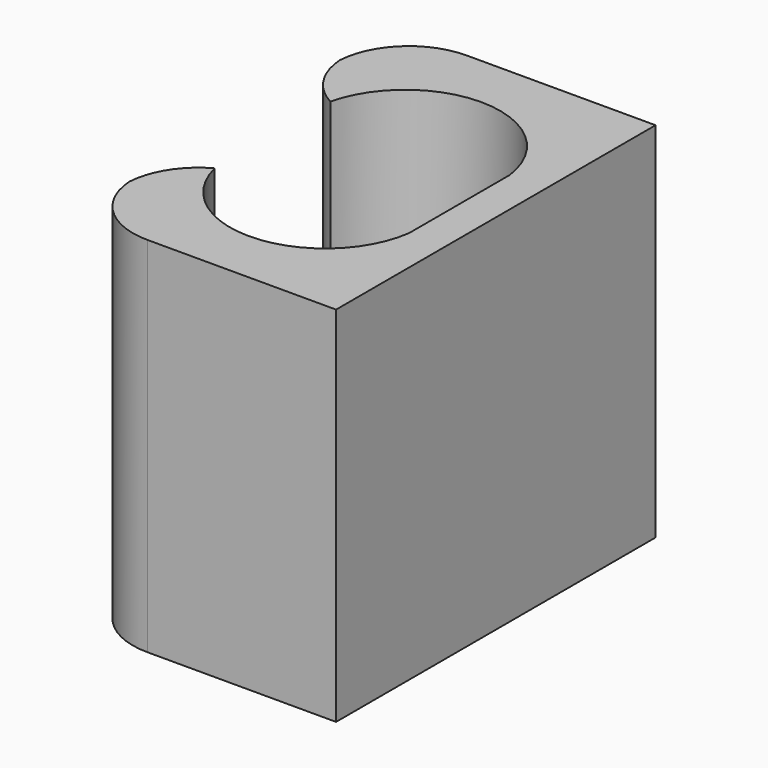
from build123d import *

# Parameters (mm, degrees)
F1_DEPTH    = 10
F2_DEPTH    = 5
F3_T1_DEPTH = 20


# Not quite as in the source:
# - a fillet or chamfer that OpenCascade refuses, or shapes differently, is made with other operations: its cross-section is extruded or revolved along the edge and cut away or added


with BuildPart() as f1:
    # F0 (on Top) → F1 (new body)
    with BuildSketch(Plane.XY):
        with BuildLine():
            ThreePointArc((-2.8424912948, 2.0151155274), (-0.2360435678, 4.2655420814), (2.3550239983, 1.9974242942))
            Line((2.3550239983, 1.9974242942), (2.3550239983, -1.4671932394))
            ThreePointArc((2.3550239983, -1.4671932394), (-0.2360435678, -3.7353110266), (-2.8424912948, -1.4848844726))
            Line((-2.8424912948, -1.4848844726), (-3.8449760017, -1.4848844726))
            Line((-3.8449760017, -1.4848844726), (-3.8449760017, -5.2353262286))
            Line((-3.8449760017, -5.2353262286), (3.3550239983, -5.2353262286))
            Line((3.3550239983, -5.2353262286), (3.3550239983, 5.7655572834))
            Line((3.3550239983, 5.7655572834), (-3.8449760017, 5.7655572834))
            Line((-3.8449760017, 5.7655572834), (-3.8449760017, 2.0151155274))
            Line((-3.8449760017, 2.0151155274), (-2.8424912948, 2.0151155274))
        make_face()
    extrude(amount=F1_DEPTH)

    # F0 (on Top) → F2 (join)
    with BuildSketch(Plane.XY):
        with BuildLine():
            Line((2.3550239983, -1.4671932394), (2.3550239983, 1.9974242942))
            ThreePointArc((2.3550239983, 1.9974242942), (-0.2360435678, 4.2655420814), (-2.8424912948, 2.0151155274))
            Line((-2.8424912948, 2.0151155274), (-1.4057946783, 2.0151155274))
            ThreePointArc((-1.4057946783, 2.0151155274), (0.7480700142, 2.1154829532), (1.8550239983, 0.2651155274))
            ThreePointArc((1.8550239983, 0.2651155274), (0.7480700142, -1.5852518984), (-1.4057946783, -1.4848844726))
            Line((-1.4057946783, -1.4848844726), (-2.8424912948, -1.4848844726))
            ThreePointArc((-2.8424912948, -1.4848844726), (-0.2360435678, -3.7353110266), (2.3550239983, -1.4671932394))
        make_face()
    extrude(amount=F2_DEPTH)

    # F3: fillet of radius 2 on 4 edges, made by hand

    # F3_s2 → F3_t1 (cut)
    with BuildSketch(Plane.XY.offset(-5)):
        with BuildLine():
            ThreePointArc((-1.8449760017, 2.0151155274), (-3.259189564, 2.600901965), (-3.8449760017, 4.0151155274))
            Line((-3.8449760017, 4.0151155274), (-3.8449760017, 2.0151155274))
            Line((-3.8449760017, 2.0151155274), (-1.8449760017, 2.0151155274))
        make_face()
        with BuildLine():
            ThreePointArc((-1.8449760017, -1.4848844726), (-3.259189564, -2.0706709102), (-3.8449760017, -3.4848844726))
            Line((-3.8449760017, -3.4848844726), (-3.8449760017, -1.4848844726))
            Line((-3.8449760017, -1.4848844726), (-1.8449760017, -1.4848844726))
        make_face()
        with BuildLine():
            ThreePointArc((-1.8449760017, -5.2353262286), (-3.259189564, -4.6495397909), (-3.8449760017, -3.2353262286))
            Line((-3.8449760017, -3.2353262286), (-3.8449760017, -5.2353262286))
            Line((-3.8449760017, -5.2353262286), (-1.8449760017, -5.2353262286))
        make_face()
        with BuildLine():
            ThreePointArc((-1.8449760017, 5.7655572834), (-3.259189564, 5.1797708458), (-3.8449760017, 3.7655572834))
            Line((-3.8449760017, 3.7655572834), (-3.8449760017, 5.7655572834))
            Line((-3.8449760017, 5.7655572834), (-1.8449760017, 5.7655572834))
        make_face()
    extrude(amount=F3_T1_DEPTH, mode=Mode.SUBTRACT)


solid = f1.part
